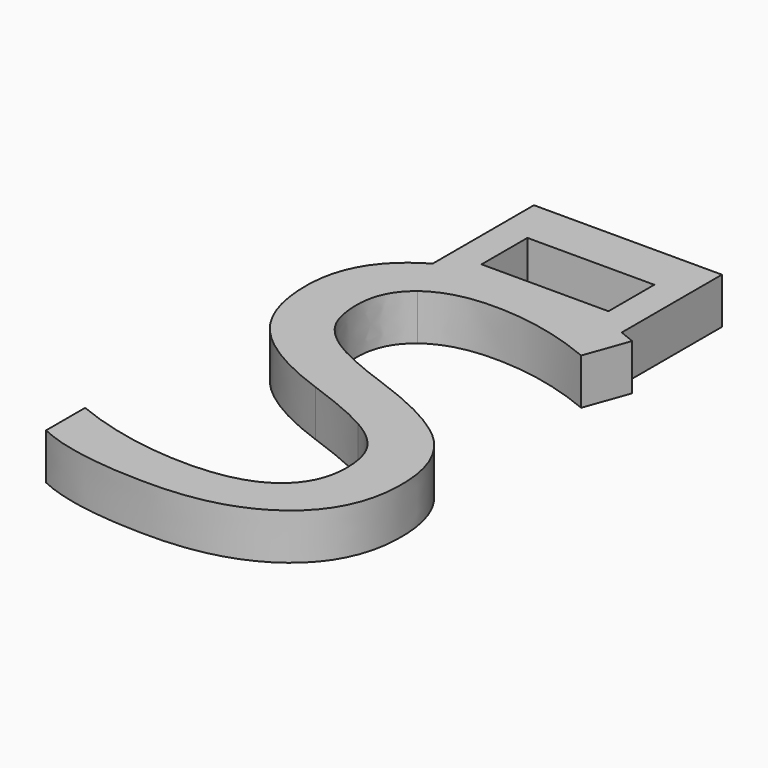
from build123d import *

# Parameters (mm, degrees)
F1_DEPTH = 2


# Not quite as in the source:
# - a feature names something its author has since deleted; it is built from what else it names


with BuildPart() as f1:
    # F0 (on Top) → F1 (new body)
    with BuildSketch(Plane.XY):
        with BuildLine():
            Line((12.1336504817, -0.6587872652), (12.1336504817, -1.7344431253))
            Line((12.1336504817, -1.7344431253), (8.0481928308, -1.7344431253))
            Line((8.0481928308, -1.7344431253), (3.9627351798, -1.7344431253))
            Line((3.9627351798, -1.7344431253), (3.9627351798, -0.7203246705))
            add(Edge.make_bspline(
                [(3.2622219629, -1.1868274189), (3.5910961238, -0.9276264724), (3.9627351798, -0.7203246705)],
                knots=[0, 0, 0, 0.2002274501, 0.2002274501, 0.2002274501], degree=2))
            add(Edge.make_bspline(
                [(1.6197190952, -4.668602098), (1.6197190952, -2.4813599438), (3.2622219629, -1.1868274189)],
                knots=[0, 0, 0, 1, 1, 1], degree=2))
            add(Edge.make_bspline(
                [(2.7526939611, -8.0468141751), (1.6197190952, -6.7522816502), (1.6197190952, -4.668602098)],
                knots=[0, 0, 0, 1, 1, 1], degree=2))
            add(Edge.make_bspline(
                [(6.5244439258, -10.2858376303), (3.8856688269, -9.3413467001), (2.7526939611, -8.0468141751)],
                knots=[0, 0, 0, 1, 1, 1], degree=2))
            add(Edge.make_bspline(
                [(9.339275448, -11.4892350655), (8.4134257862, -10.9569232912), (6.5244439258, -10.2858376303)],
                knots=[0, 0, 0, 1, 1, 1], degree=2))
            add(Edge.make_bspline(
                [(10.6607342495, -12.6491362079), (10.2651251099, -12.0215468398), (9.339275448, -11.4892350655)],
                knots=[0, 0, 0, 1, 1, 1], degree=2))
            add(Edge.make_bspline(
                [(11.0563433891, -14.2584990429), (11.0563433891, -13.276725576), (10.6607342495, -12.6491362079)],
                knots=[0, 0, 0, 1, 1, 1], degree=2))
            add(Edge.make_bspline(
                [(9.9420097917, -16.5845150837), (11.0563433891, -15.7498005116), (11.0563433891, -14.2584990429)],
                knots=[0, 0, 0, 1, 1, 1], degree=2))
            add(Edge.make_bspline(
                [(6.6280065278, -17.4192296558), (8.8276761942, -17.4192296558), (9.9420097917, -16.5845150837)],
                knots=[0, 0, 0, 1, 1, 1], degree=2))
            add(Edge.make_bspline(
                [(3.9105238514, -17.1333968743), (5.2816927018, -17.4192296558), (6.6280065278, -17.4192296558)],
                knots=[0, 0, 0, 1, 1, 1], degree=2))
            add(Edge.make_bspline(
                [(1.3711688504, -16.3587486114), (2.539355001, -16.8475640928), (3.9105238514, -17.1333968743)],
                knots=[0, 0, 0, 1, 1, 1], degree=2))
            Line((1.3711688504, -16.3587486114), (1.3711688504, -18.4797107003))
            add(Edge.make_bspline(
                [(6.5492989503, -19.349636557), (3.1855856374, -19.349636557), (1.3711688504, -18.4797107003)],
                knots=[0, 0, 0, 1, 1, 1], degree=2))
            add(Edge.make_bspline(
                [(11.4685225451, -17.949470178), (9.6561770102, -19.349636557), (6.5492989503, -19.349636557)],
                knots=[0, 0, 0, 1, 1, 1], degree=2))
            add(Edge.make_bspline(
                [(13.28086808, -14.0513738389), (13.28086808, -16.549303799), (11.4685225451, -17.949470178)],
                knots=[0, 0, 0, 1, 1, 1], degree=2))
            add(Edge.make_bspline(
                [(12.1623919785, -10.89478573), (13.28086808, -12.1126819295), (13.28086808, -14.0513738389)],
                knots=[0, 0, 0, 1, 1, 1], degree=2))
            add(Edge.make_bspline(
                [(8.0654554435, -8.6164084861), (11.0439158769, -9.6768895306), (12.1623919785, -10.89478573)],
                knots=[0, 0, 0, 1, 1, 1], degree=2))
            add(Edge.make_bspline(
                [(5.4308228487, -7.4585785958), (6.2924636973, -7.9826053619), (8.0654554435, -8.6164084861)],
                knots=[0, 0, 0, 1, 1, 1], degree=2))
            add(Edge.make_bspline(
                [(4.2067128931, -6.3048912095), (4.5691820001, -6.9345518297), (5.4308228487, -7.4585785958)],
                knots=[0, 0, 0, 1, 1, 1], degree=2))
            add(Edge.make_bspline(
                [(3.8442437861, -4.6934571225), (3.8442437861, -5.6752305894), (4.2067128931, -6.3048912095)],
                knots=[0, 0, 0, 1, 1, 1], degree=2))
            add(Edge.make_bspline(
                [(4.8280885051, -2.6097775703), (3.8442437861, -3.3595708088), (3.8442437861, -4.6934571225)],
                knots=[0, 0, 0, 1, 1, 1], degree=2))
            add(Edge.make_bspline(
                [(7.5600699457, -1.8599843319), (5.811933224, -1.8599843319), (4.8280885051, -2.6097775703)],
                knots=[0, 0, 0, 1, 1, 1], degree=2))
            add(Edge.make_bspline(
                [(12.1168244336, -2.8417577988), (9.7721671244, -1.8599843319), (7.5600699457, -1.8599843319)],
                knots=[0, 0, 0, 1, 1, 1], degree=2))
            Line((12.1168244336, -2.8417577988), (12.8044801109, -0.9279209139))
            add(Edge.make_bspline(
                [(12.1336504817, -0.6587872652), (12.4734710603, -0.7832491261), (12.8044801109, -0.9279209139)],
                knots=[0.8603049894, 0.8603049894, 0.8603049894, 1, 1, 1], degree=2))
        make_face()
        with BuildLine():
            Line((8.0481928308, -1.7344431253), (12.1336504817, -1.7344431253))
            Line((12.1336504817, -1.7344431253), (12.1336504817, -0.6587872652))
            add(Edge.make_bspline(
                [(8.0481928308, 0.1014929313), (10.2292854005, 0.0387008703), (12.1336504817, -0.6587872652)],
                knots=[0.0774498097, 0.0774498097, 0.0774498097, 0.8603049894, 0.8603049894, 0.8603049894], degree=2))
            Line((8.0481928308, 0.1014929313), (8.0481928308, -1.7344431253))
        make_face()
        with BuildLine():
            Line((3.9627351798, -1.7344431253), (8.0481928308, -1.7344431253))
            Line((8.0481928308, -1.7344431253), (8.0481928308, 0.1014929313))
            add(Edge.make_bspline(
                [(7.6139224988, 0.1077051061), (7.8324119189, 0.1077051061), (8.0481928308, 0.1014929313)],
                knots=[0, 0, 0, 0.0774498097, 0.0774498097, 0.0774498097], degree=2))
            add(Edge.make_bspline(
                [(3.9627351798, -0.7203246705), (5.4471805714, 0.1077051061), (7.6139224988, 0.1077051061)],
                knots=[0.2002274501, 0.2002274501, 0.2002274501, 1, 1, 1], degree=2))
            Line((3.9627351798, -0.7203246705), (3.9627351798, -1.7344431253))
        make_face()
        with BuildLine():
            add(Edge.make_bspline(
                [(8.0481928308, 0.1014929313), (10.2292854005, 0.0387008703), (12.1336504817, -0.6587872652)],
                knots=[0.0774498097, 0.0774498097, 0.0774498097, 0.8603049894, 0.8603049894, 0.8603049894], degree=2))
            Line((12.1336504817, -0.6587872652), (12.1336504817, 3.1816535629))
            Line((12.1336504817, 3.1816535629), (12.1336504817, 4.784271121))
            Line((12.1336504817, 4.784271121), (8.0481928308, 4.784271121))
            Line((8.0481928308, 4.784271121), (8.0481928308, 2.7708526759))
            Line((8.0481928308, 2.7708526759), (10.8064850792, 2.7708526759))
            Line((10.8064850792, 2.7708526759), (10.8064850792, 0.2789753198))
            Line((10.8064850792, 0.2789753198), (8.0481928308, 0.2789753198))
            Line((8.0481928308, 0.2789753198), (8.0481928308, 0.1014929313))
        make_face()
        with BuildLine():
            add(Edge.make_bspline(
                [(7.6139224988, 0.1077051061), (7.8324119189, 0.1077051061), (8.0481928308, 0.1014929313)],
                knots=[0, 0, 0, 0.0774498097, 0.0774498097, 0.0774498097], degree=2))
            Line((8.0481928308, 0.1014929313), (8.0481928308, 0.2789753198))
            Line((8.0481928308, 0.2789753198), (5.2899005823, 0.2789753198))
            Line((5.2899005823, 0.2789753198), (5.2899005823, 2.7708526759))
            Line((5.2899005823, 2.7708526759), (8.0481928308, 2.7708526759))
            Line((8.0481928308, 2.7708526759), (8.0481928308, 4.784271121))
            Line((8.0481928308, 4.784271121), (3.9627351798, 4.784271121))
            Line((3.9627351798, 4.784271121), (3.9627351798, 3.1816535629))
            Line((3.9627351798, 3.1816535629), (3.9627351798, -0.7203246705))
            add(Edge.make_bspline(
                [(3.9627351798, -0.7203246705), (5.4471805714, 0.1077051061), (7.6139224988, 0.1077051061)],
                knots=[0.2002274501, 0.2002274501, 0.2002274501, 1, 1, 1], degree=2))
        make_face()
    extrude(amount=F1_DEPTH)


solid = f1.part
